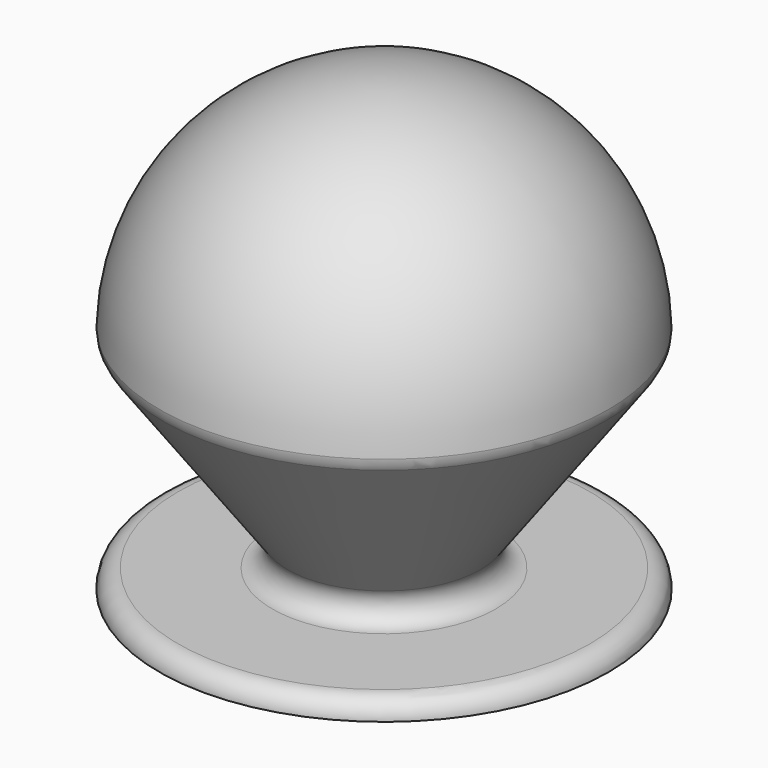
from build123d import *

# Parameters (mm, degrees)
F2_R = 4.99999
F3_R = 5


# Not quite as in the source:
# - a fillet or chamfer is up to 0.001 mm smaller than in the source, because OpenCascade refuses the exact size


with BuildPart() as f1:
    # F0 (on Front) → F1 (revolve)
    with BuildSketch(Plane.XZ):
        with BuildLine():
            Line((0, 120), (0, 0))
            Line((0, 0), (60, 0))
            Line((60, 0), (60, 5))
            Line((60, 5), (20, 5))
            Line((20, 5), (60, 60))
            ThreePointArc((60, 60), (42.4264068712, 102.4264068712), (0, 120))
        make_face()
    revolve(axis=Axis((0, 0, 60), (0, 0, -1)))

    # F2 (radius 5 in the source; OpenCascade refuses exactly that, so slightly less here)
    f2_edges = [f1.edges().sort_by_distance(p)[0] for p in [
        (-60, 0, 5),
        (-20, 0, 5),
    ]]
    fillet(f2_edges, radius=F2_R)

    # F3
    f3_edges = [f1.edges().sort_by_distance(p)[0] for p in [
        (-60, 0, 60),
    ]]
    fillet(f3_edges, radius=F3_R)


solid = f1.part
